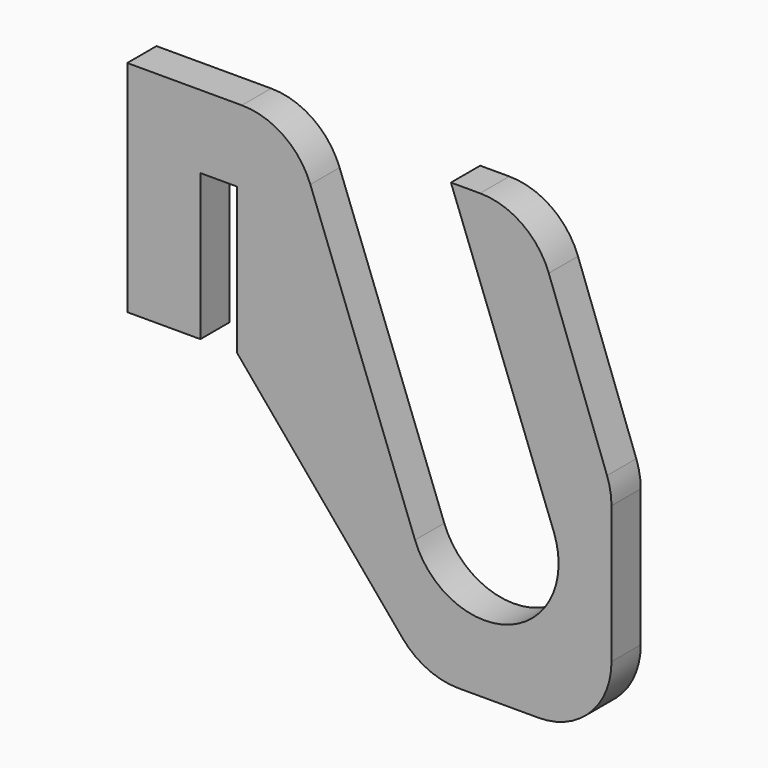
from build123d import *

# Parameters (mm, degrees)
F1_DEPTH = 3.175


# Not quite as in the source:
# - a length typed as a fraction of an inch, garbled in the dataset ("3 / 203.2 mm" for 3/8 in), is restored


with BuildPart() as f1:
    # F0 (on Front) → F1 (new body)
    with BuildSketch(Plane.XZ):
        with BuildLine():
            Line((0, 19.05), (0, 0))
            Line((0, 0), (6.35, 0))
            Line((6.35, 0), (6.35, 12.7))
            Line((6.35, 12.7), (9.525, 12.7))
            Line((9.525, 12.7), (9.525, 0))
            Line((9.525, 0), (23.8846407704, -17.1268223527))
            ThreePointArc((23.8846407704, -17.1268223527), (26.0658700781, -18.8015604613), (28.7506271903, -19.3970336129))
            Line((28.7506271903, -19.3970336129), (35.7011077573, -19.3970336129))
            ThreePointArc((35.7011077573, -19.3970336129), (40.1912358178, -17.5371616734), (42.0511077573, -13.0470336129))
            Line((42.0511077573, -13.0470336129), (42.0511077573, -1.1253461624))
            ThreePointArc((42.0511077573, -1.1253461624), (41.9536799226, -0.017266148), (41.6643860823, 1.0568113981))
            Line((41.6643860823, 1.0568113981), (36.6052420996, 14.8821575605))
            ThreePointArc((36.6052420996, 14.8821575605), (34.2796690603, 17.9047670702), (30.6419637747, 19.05))
            Line((30.6419637747, 19.05), (28.1090781347, 19.05))
            Line((28.1090781347, 19.05), (37.0488404527, -4.7744145618))
            ThreePointArc((37.0488404527, -4.7744145618), (33.2823465228, -13.0652413354), (24.9915197492, -9.2987474054))
            Line((24.9915197492, -9.2987474054), (15.8997145825, 14.9308604634))
            ThreePointArc((15.8997145825, 14.9308604634), (13.5708732383, 17.9196007483), (9.9544844278, 19.05))
            Line((9.9544844278, 19.05), (0, 19.05))
        make_face()
    extrude(amount=F1_DEPTH)


solid = f1.part
